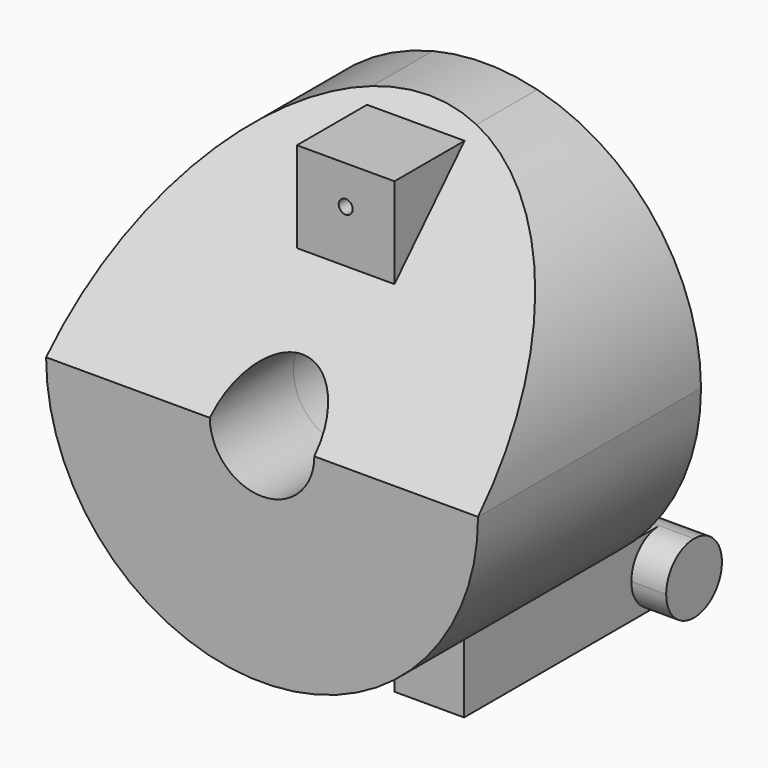
from build123d import *

# Parameters (mm, degrees)
F1_DEPTH       = 40
F3_DEPTH       = 44.8
F3_DEPTH_BACK  = 52.7
F5_DEPTH       = 25
F6_DEPTH       = 25
F7_DEPTH       = 41
F8_W           = 5
F8_H           = 10
F9_DEPTH       = 10
F10_DEPTH      = 30
F12_DEPTH      = 25
F13_DEPTH      = 5
F13_DEPTH_BACK = 15


with BuildPart() as f1:
    # F0 (on Front) → F1 (new body)
    with BuildSketch(Plane.XZ):
        with BuildLine():
            ThreePointArc((-7.5, 30.079062), (-19.085335, -24.428467), (31, 0))
            ThreePointArc((31, 0), (24.428467, 19.085335), (7.5, 30.079062))
            Line((7.5, 30.079062), (7.5, 0))
            ThreePointArc((7.5, 0), (0, -7.5), (-7.5, 0))
            Line((-7.5, 0), (-7.5, 30.079062))
        make_face()
        with BuildLine():
            Line((7.5, 0), (7.5, 30.079062))
            ThreePointArc((7.5, 30.079062), (0, 31), (-7.5, 30.079062))
            Line((-7.5, 30.079062), (-7.5, 0))
            ThreePointArc((-7.5, 0), (0, 7.5), (7.5, 0))
        make_face()
    extrude(amount=F1_DEPTH)

    # F2 (on Right) → F3 (cut, two sides)
    with BuildSketch(Plane.YZ) as f3_sk:
        Polygon((-40, 0), (-10, 31), (-40, 31), align=None)
    extrude(amount=F3_DEPTH, mode=Mode.SUBTRACT)
    extrude(f3_sk.sketch, amount=-F3_DEPTH_BACK, mode=Mode.SUBTRACT)

    # F4 (on Front) → F5 (cut)
    with BuildSketch(Plane.XZ):
        with BuildLine():
            ThreePointArc((1, 23), (-0.707107, 23.707107), (0, 22))
            ThreePointArc((0, 22), (0.707107, 22.292893), (1, 23))
        make_face()
    extrude(amount=F5_DEPTH, mode=Mode.SUBTRACT)

    # F4 (on Front) → F6 (join)
    with BuildSketch(Plane.XZ):
        with BuildLine():
            ThreePointArc((-7, 2.692582), (-4.245918, 6.182409), (0, 7.5))
            Line((0, 7.5), (0, 11.5))
            Line((0, 11.5), (-7, 11.5))
            Line((-7, 11.5), (-7, 2.692582))
        make_face()
        with BuildLine():
            Line((0, 11.5), (0, 7.5))
            ThreePointArc((0, 7.5), (4.245918, 6.182409), (7, 2.692582))
            Line((7, 2.692582), (7, 11.5))
            Line((7, 11.5), (0, 11.5))
        make_face()
        with BuildLine():
            ThreePointArc((7, 2.692582), (4.245918, 6.182409), (0, 7.5))
            ThreePointArc((0, 7.5), (-4.245918, 6.182409), (-7, 2.692582))
            ThreePointArc((-7, 2.692582), (-1.369306, -7.373941), (7.5, 0))
            ThreePointArc((7.5, 0), (7.373941, 1.369306), (7, 2.692582))
        make_face()
        Polygon((-7, 11.5), (0, 11.5), (7, 11.5), (7, 28.5), (-7, 28.5), align=None)
        with BuildLine():
            ThreePointArc((1, 23), (0.707107, 22.292893), (0, 22))
            ThreePointArc((0, 22), (-0.707107, 23.707107), (1, 23))
        make_face(mode=Mode.SUBTRACT)
    extrude(amount=F6_DEPTH)

    # F7 (cut): a face of the model
    f7_faces = [f1.faces().sort_by_distance(p)[0] for p in [
        (0, -25, 0),
    ]]
    extrude(f7_faces, amount=-F7_DEPTH, mode=Mode.SUBTRACT)

    # F8 (on Front) → F9 (join)
    with BuildSketch(Plane.XZ):
        with BuildLine():
            Line((5, -36), (5, -10.356158))
            ThreePointArc((5, -10.356158), (0, -11.5), (-5, -10.356158))
            Line((-5, -10.356158), (-5, -36))
            Line((-5, -36), (0, -36))
            Line((0, -36), (5, -36))
        make_face()
        with Locations((2.5, -41)):
            Rectangle(F8_W, F8_H)
        with Locations((-2.5, -41)):
            Rectangle(F8_W, F8_H)
    extrude(amount=F9_DEPTH)

    # F8 (on Front) → F10 (join)
    with BuildSketch(Plane.XZ):
        with Locations((2.5, -41)):
            Rectangle(F8_W, F8_H)
        with Locations((-2.5, -41)):
            Rectangle(F8_W, F8_H)
    extrude(amount=-F10_DEPTH)

    # F11 (on face) → F12 (cut)
    with BuildSketch(Plane.YZ.offset(5)):
        with BuildLine():
            Line((30, -36), (25, -36))
            ThreePointArc((25, -36), (28.535534, -37.464466), (30, -41))
            Line((30, -41), (30, -36))
        make_face()
        with BuildLine():
            Line((30, -46), (30, -41))
            ThreePointArc((30, -41), (28.535534, -44.535534), (25, -46))
            Line((25, -46), (30, -46))
        make_face()
    extrude(amount=-F12_DEPTH, mode=Mode.SUBTRACT)

    # F11 (on face) → F13 (join, two sides)
    with BuildSketch(Plane.YZ.offset(5)) as f13_sk:
        with BuildLine():
            Line((30, -41), (20, -41))
            ThreePointArc((20, -41), (21.464466, -44.535534), (25, -46))
            ThreePointArc((25, -46), (28.535534, -44.535534), (30, -41))
        make_face()
        with BuildLine():
            ThreePointArc((30, -41), (28.535534, -37.464466), (25, -36))
            ThreePointArc((25, -36), (21.464466, -37.464466), (20, -41))
            Line((20, -41), (30, -41))
        make_face()
    extrude(amount=F13_DEPTH)
    extrude(f13_sk.sketch, amount=-F13_DEPTH_BACK)


solid = f1.part
